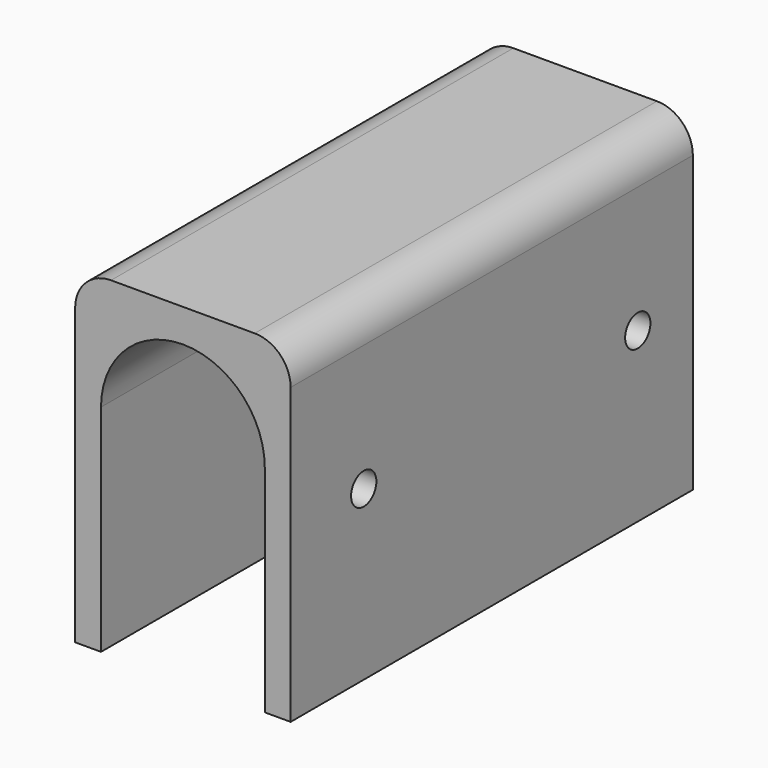
from build123d import *

# Parameters (mm, degrees)
F0_W     = 30
F0_H     = 46
F1_DEPTH = 70
F2_W     = 22.8
F2_H     = 30
F3_DEPTH = 70
F4_R     = 2.2
F5_DEPTH = 3.6
F6_R     = 5


# Not quite as in the source:
# - a feature names something its author has since deleted; it is built from what else it names


with BuildPart() as f1:
    # F0 (on Front) → F1 (new body)
    with BuildSketch(Plane.XZ):
        with Locations((-35.3317022547, -0.4139923602)):
            Rectangle(F0_W, F0_H)
    extrude(amount=F1_DEPTH)

    # F2 (on face) → F3 (cut, through all)
    with BuildSketch(Plane.XZ.offset(70)):
        with Locations((-35.3317022547, -8.4139923602)):
            Rectangle(F2_W, F2_H)
        with BuildLine():
            ThreePointArc((-23.9317022547, 6.5860076398), (-35.3317022547, 17.9860076398), (-46.7317022547, 6.5860076398))
            Line((-46.7317022547, 6.5860076398), (-23.9317022547, 6.5860076398))
        make_face()
    extrude(amount=-F3_DEPTH, mode=Mode.SUBTRACT)

    # F4 (on face) → F5 (cut, through all)
    with BuildSketch(Plane.YZ.offset(-20.3317022547)):
        with Locations((-9.5844314775, 0)):
            Circle(F4_R)
        with Locations((-57.2790902557, 0)):
            Circle(F4_R)
    extrude(amount=-F5_DEPTH, mode=Mode.SUBTRACT)

    # F6
    f6_edges = [f1.edges().sort_by_distance(p)[0] for p in [
        (-20.331702, -35, 22.586008),
        (-50.331702, -35, 22.586008),
    ]]
    fillet(f6_edges, radius=F6_R)


solid = f1.part
